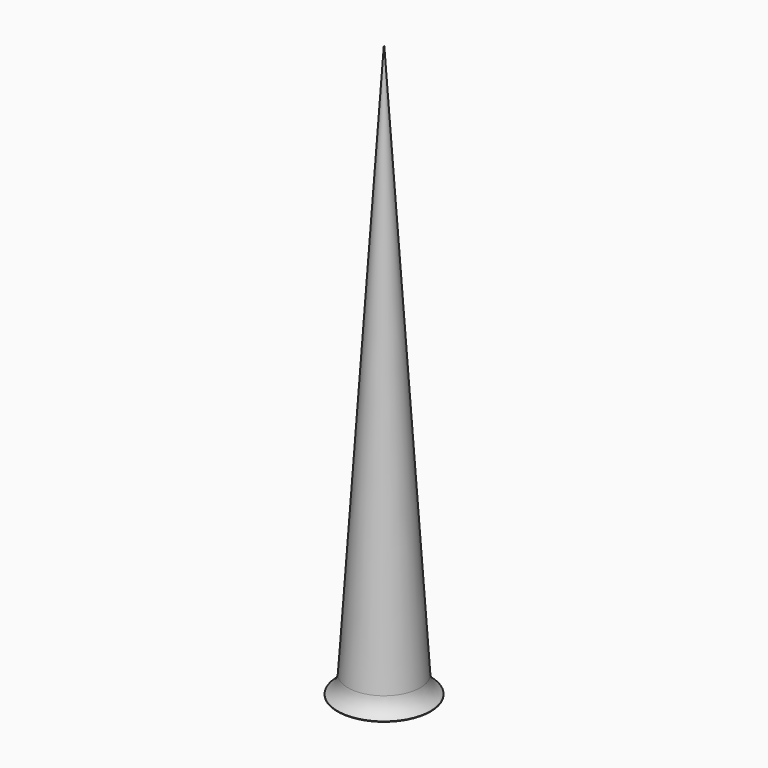
from build123d import *

# Parameters (mm, degrees)
F0_R     = 85
F2_R     = 0.5
F4_R     = 105.9677495378
F5_DEPTH = 1


# Not quite as in the source:
# - a fillet or chamfer that OpenCascade refuses, or shapes differently, is made with other operations: its cross-section is extruded or revolved along the edge and cut away or added


with BuildPart() as f3:
    # F0 (on Top) → F3 section 0
    with BuildSketch(Plane.XY):
        Circle(F0_R)
    # F2 (on offset) → F3 section 1
    with BuildSketch(Plane.XY.offset(1300)):
        Circle(F2_R)
    loft()

    # F4 (on Top) → F5 (join)
    with BuildSketch(Plane.XY):
        Circle(F4_R)
    extrude(amount=F5_DEPTH)

    # F6: fillet of radius 50 on 1 edges, made by hand


with BuildPart() as f6_tool2:
    # F6_s3 → F6_t4 (revolve)
    with BuildSketch(Plane.XZ):
        with BuildLine():
            ThreePointArc((105.9675390616, 0.9996598533), (89.4115983215, 17.7775955554), (82.3816590809, 40.2760011541))
            Line((82.3816590809, 40.2760011541), (77.3920405677, 39.9516759507))
            ThreePointArc((77.3920405677, 39.9516759507), (78.6689106061, 20.3136883463), (79.9453814868, 0.6756747966))
            Line((79.9453814868, 0.6756747966), (84.935, -4.0001479723))
            ThreePointArc((84.935, -4.0001479723), (95.4512695308, -4.0001479723), (103.3365085465, -3.2522994801))
            Line((103.3365085465, -3.2522994801), (105.9675390616, 0.9996598533))
        make_face()
    revolve(axis=Axis((0, 0, 1), (0, 0, 1)))

    split(bisect_by=Plane.XY, keep=Keep.TOP)


with BuildPart() as f3_1:
    add(f3.part)

    # F6_t1: union F6_tool2
    add(f6_tool2.part)


solid = f3_1.part
